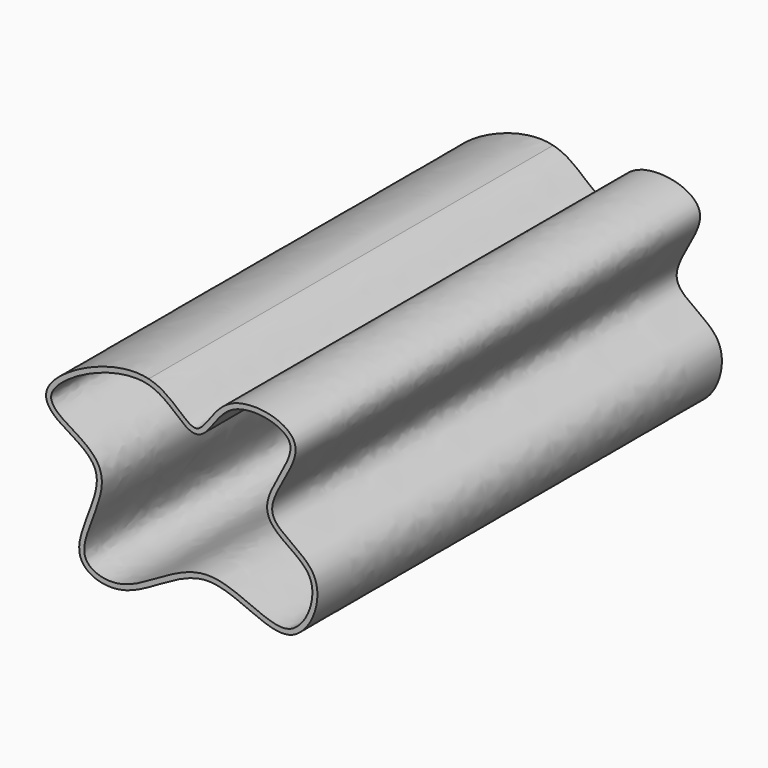
from build123d import *

# Parameters (mm, degrees)
F1_DEPTH = 254
F2_T     = -2.54


with BuildPart() as f1:
    # F0 (on Front) → F1 (new body)
    with BuildSketch(Plane.XZ):
        with BuildLine():
            add(Edge.make_bspline(
                [(14.972730386, 40.1406101882), (11.0393549573, 35.458290892), (4.3975166084, 22.3087954161), (-6.444831778, 41.2649562059), (-18.4429828078, 44.2089177668)],
                knots=[0.8852065932, 0.8852065932, 0.8852065932, 0.8852065932, 0.928553384, 1, 1, 1, 1], degree=3))
            add(Edge.make_bspline(
                [(-18.4429828078, 44.2089177668), (-35.094000229, 48.2945435534), (-75.4039068495, 28.7627119174), (-67.0210177787, 9.5224148903), (-32.240300341, -2.6203459485), (-64.7104835314, -47.4681039556), (-27.1916495635, -60.7914709336), (9.830150405, -21.1776329246), (54.941729477, -61.5304587528), (76.0521080016, -10.2479448183), (28.2811395171, 1.0900838977), (72.2426421397, 44.0768640266), (28.0295814463, 53.219341033), (17.0690015243, 42.6360269058), (14.972730386, 40.1406101882)],
                knots=[0, 0, 0, 0, 0.0991535149, 0.1493467633, 0.2204507163, 0.3047843999, 0.3706708885, 0.4633927027, 0.5518487194, 0.6284660124, 0.7034041754, 0.7839698521, 0.8621051557, 0.8852065932, 0.8852065932, 0.8852065932, 0.8852065932], degree=3))
        make_face()
    extrude(amount=F1_DEPTH)

    # F2
    f2_openings = [f1.faces().sort_by_distance(p)[0] for p in [
        (-0.349926, -254, -1.204363),
    ]]
    offset(amount=F2_T, openings=f2_openings, kind=Kind.INTERSECTION)


solid = f1.part
